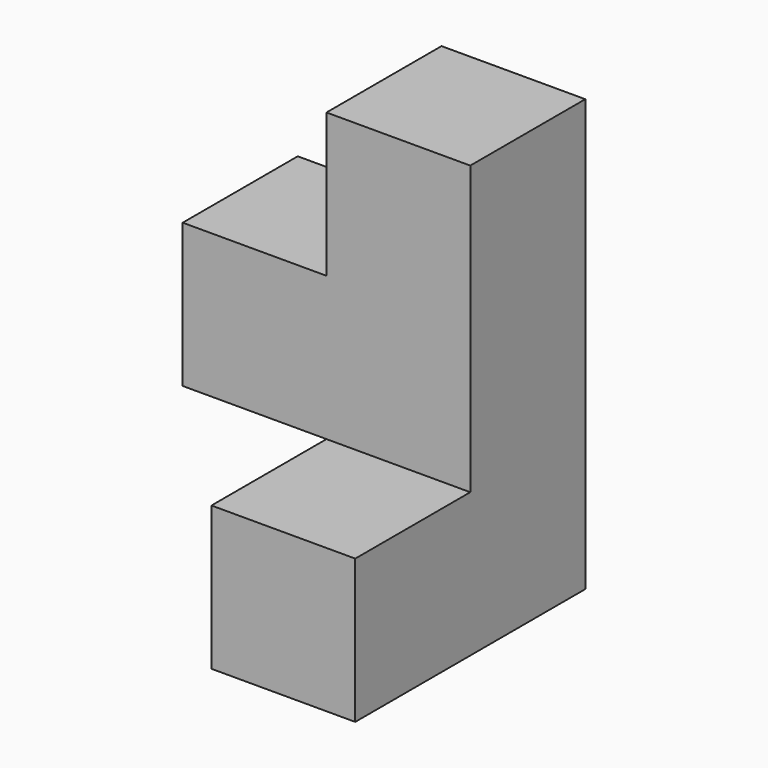
from build123d import *

# Parameters (mm, degrees)
F1_W     = 76.2
F1_H     = 76.2
F2_DEPTH = 228.6
F3_W     = 76.2
F3_H     = 76.2
F4_DEPTH = 76.2
F5_W     = 76.2
F5_H     = 76.2
F6_DEPTH = 76.2


# Not quite as in the source:
# - a variable given as a bare number and used for a length is read in inches; the dataset says mm whatever the document's units were


with BuildPart() as f2:
    # F1 (on Top) → F2 (new body)
    with BuildSketch(Plane.XY):
        Rectangle(F1_W, F1_H)
    extrude(amount=F2_DEPTH)

    # F3 (on face) → F4 (join)
    with BuildSketch(Plane.XZ.offset(38.1)):
        with Locations((0, 38.1)):
            Rectangle(F3_W, F3_H)
    extrude(amount=F4_DEPTH)

    # F5 (on face) → F6 (join)
    with BuildSketch(Plane(origin=(-38.1, 0, 0), x_dir=(0, -1, 0), z_dir=(-1, 0, 0))):
        with Locations((0, 114.3)):
            Rectangle(F5_W, F5_H)
    extrude(amount=F6_DEPTH)


solid = f2.part
